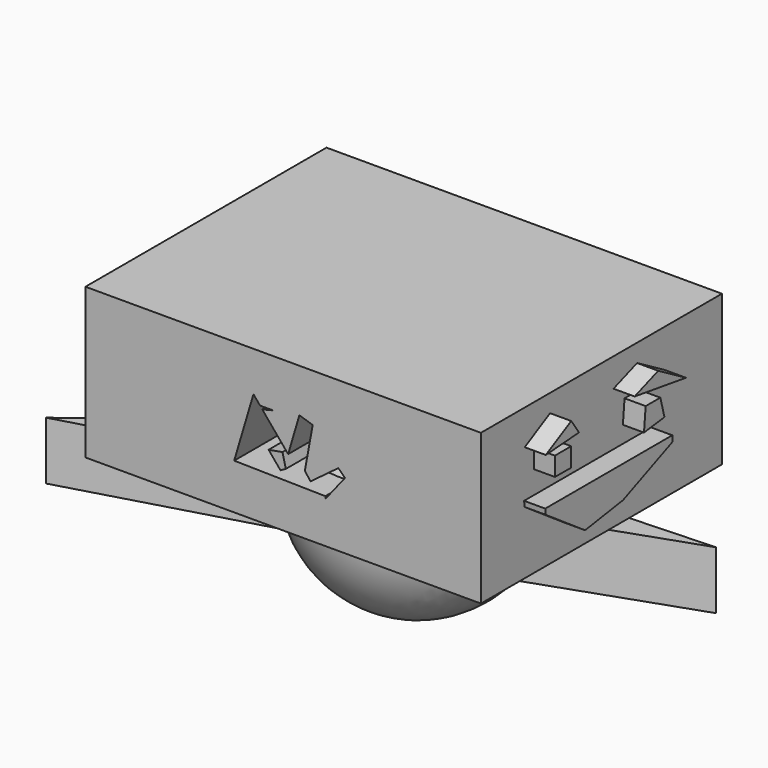
from build123d import *

# Parameters (mm, degrees)
F0_W      = 145.4915776849
F0_H      = 129.8910155892
F1_DEPTH  = 64.8
F5_DEPTH  = 9.1
F7_DEPTH  = 194.8
F8_W      = 129.8910155892
F8_H      = 64.8
F9_DEPTH  = 25
F11_DEPTH = 25


with BuildPart() as f1:
    # F0 (on Top) → F1 (new body)
    with BuildSketch(Plane.XY):
        with Locations((-0.2166293561, 8.3162896335)):
            Rectangle(F0_W, F0_H)
    extrude(amount=F1_DEPTH)

    # F4 (on face) → F5 (join)
    with BuildSketch(Plane.YZ.offset(72.5291594863)):
        Polygon((-19.3242635578, 47.511447221), (-28.1233321875, 47.511447221), (-28.1233321875, 39.4137501717), (-19.3242635578, 39.3499881029), align=None)
        Polygon((28.6880470812, 46.4275032282), (20.7816362381, 46.4275032282), (19.8889784515, 36.7357730865), (30.919695273, 38.1385236979), align=None)
        Polygon((-33.3491843987, 29.5307394117), (-33.0329574645, 27.0440466702), (-11.8641834706, 12.5702153891), (8.6032152176, 15.6945213675), (35.1279452443, 26.9165225327), (35.1279452443, 29.5307394117), (-3.3201600891, 29.5307394117), align=None)
        Polygon((27.5403410196, 57.0756494999), (14.8518308997, 52.4848327041), (42.5242660567, 48.3403429389), align=None)
        Polygon((-19.3242635578, 57.0756494999), (-33.0329574645, 49.7430935502), (-15.1160135865, 51.018320024), align=None)
    extrude(amount=F5_DEPTH)

    # F6 (on face) → F7 (cut)
    with BuildSketch(Plane.XZ.offset(56.6292181611)):
        Polygon((11.0493209213, 31.4134769142), (-0.9407399921, 22.4588736892), (-3.3654462761, 25.7055140274), (0, 44.1624037921), (-5.7215876877, 46.059563756), (-10.578321293, 29.6680871397), (-21.3376915526, 42.5574875524), (-21.7236716623, 43.0198800592), (-22.6773883194, 44.1624037921), (-25.5279541016, 47.5772954524), (-33.8349560351, 19.6422461394), (5.4337228648, 18.9431003046), (6.2996602968, 18.9276830162), (13.9330085367, 28.6056771874), align=None)
        Polygon((-13.0330054452, 29.6680871397), (-11.5648452193, 23.7489435822), (-13.8707014465, 22.4588736892), (-19.0017186105, 28.6056771874), align=None, mode=Mode.SUBTRACT)
        Polygon((5.4337228648, 17.829798162), (6.2996602968, 18.9276830162), (5.4337228648, 18.9431003046), align=None)
        Polygon((-22.6773883194, 44.1624037921), (-21.7236716623, 43.0198800592), (-17.1173883194, 44.1624037921), align=None)
    extrude(amount=-F7_DEPTH, mode=Mode.SUBTRACT)

    # F8 (on face) → F9 (join)
    with BuildSketch(Plane(origin=(-72.9624181986, 0, 0), x_dir=(0, -1, 0), z_dir=(-1, 0, 0))):
        with Locations((-8.3162896335, 32.4)):
            Rectangle(F8_W, F8_H)
        Polygon((-33.7973619791, 46.7837587321), (-32.2640491742, 50.7749373199), (-27.4221395057, 50.9029878243), (-14.7904808392, 51.2370482208), (-7.7179151013, 51.4240912828), (-4.7785166523, 51.5018274406), (5.8706160635, 51.7834573984), (20.7907762378, 32.7825695276), (21.4921496809, 32.7825695276), (14.9213466931, 25.4723990848), (-17.3487263283, 21.3266381618), (-20.4029875619, 11.7817013825), (-34.6178524196, 14.1642494127), (-38.7577424652, 24.4219713113), (-39.5912416279, 23.7922165543), (-39.1102442103, 25.2953918203), (-40.3563790023, 28.3830352128), (-40.8664681017, 28.3830352128), align=None, mode=Mode.SUBTRACT)
        Polygon((14.9213466931, 25.4723990848), (-7.7179151013, 51.4240912828), (-9.6287822342, 45.4523997401), (-11.6142911711, 39.2474435073), (-17.3487263283, 21.3266381618), align=None)
        Polygon((-17.3487263283, 21.3266381618), (-25.715688368, 34.2759651439), (-38.7577424652, 24.4219713113), (-34.6178524196, 14.1642494127), (-20.4029875619, 11.7817013825), align=None)
        Polygon((-4.7785166523, 51.5018274406), (-7.7179151013, 51.4240912828), (14.9213466931, 25.4723990848), (21.4921496809, 32.7825695276), (20.7907762378, 32.7825695276), (5.8706160635, 51.7834573984), align=None)
        Polygon((-14.7904808392, 51.2370482208), (-27.4221395057, 50.9029878243), (-33.7973619791, 46.7837587321), (-25.715688368, 34.2759651439), (-25.2449326217, 34.6316471696), (-11.6142911711, 39.2474435073), (-9.6287822342, 45.4523997401), align=None)
        Polygon((-25.715688368, 34.2759651439), (-33.7973619791, 46.7837587321), (-40.8664681017, 28.3830352128), (-40.3563790023, 28.3830352128), (-39.1102442103, 25.2953918203), (-38.7577424652, 24.4219713113), align=None)
        Polygon((-25.2449326217, 34.6316471696), (-25.715688368, 34.2759651439), (-17.3487263283, 21.3266381618), (-11.6142911711, 39.2474435073), align=None)
        Polygon((-7.7179151013, 51.4240912828), (-14.7904808392, 51.2370482208), (-9.6287822342, 45.4523997401), align=None)
        Polygon((-27.4221395057, 50.9029878243), (-32.2640491742, 50.7749373199), (-33.7973619791, 46.7837587321), align=None)
        Polygon((-39.5912416279, 23.7922165543), (-38.7577424652, 24.4219713113), (-39.1102442103, 25.2953918203), align=None)
    extrude(amount=F9_DEPTH)

    # F10 (on face) → F11 (join)
    with BuildSketch(Plane(origin=(0, 0, 0), x_dir=(1, 0, 0), z_dir=(0, 0, -1))):
        Polygon((-66.0155639052, -3.5001058131), (-46.312995255, 8.4308944643), (-7.864049999, 8.4308944643), (-126.4367699623, 42.253639549), align=None)
        Polygon((-7.864049999, 8.4308944643), (-46.312995255, 8.4308944643), (-66.0155639052, -3.5001058131), (-17.1969756484, -22.983757779), (-38.9792583883, -28.7850722671), (24.0689646453, -21.1229603738), (108.7900176644, -24.8445570469), align=None)
        Polygon((6.5555688925, 8.4308944643), (-7.864049999, 8.4308944643), (108.7900176644, -24.8445570469), (13.1230894476, 8.4308944643), (12.3568801209, 8.4308944643), (10.2498008637, 5.0650389167), (9.0183902066, 6.1869907659), align=None)
        Polygon((11.4812115207, 8.8900875296), (9.0183902066, 6.1869907659), (10.2498008637, 5.0650389167), (12.3568801209, 8.4308944643), align=None)
    extrude(amount=F11_DEPTH)


with BuildPart() as f3:
    # F2 (on Top) → F3 (revolve)
    with BuildSketch(Plane.XY):
        with BuildLine():
            ThreePointArc((6.9453806266, -46.5313356638), (35.6381929992, -30.7135590654), (47.0468225357, 0))
            ThreePointArc((47.0468225357, 0), (30.7436495281, 35.6122384076), (-6.8667663549, 46.5430019502))
            Line((-6.8667663549, 46.5430019502), (6.9453806266, -46.5313356638))
        make_face()
    revolve(axis=Axis((0.0393071358, 0.0058331432, 0), (-0.146791549, 0.9891674485, 0)))


solid = Compound([f1.part, f3.part])
